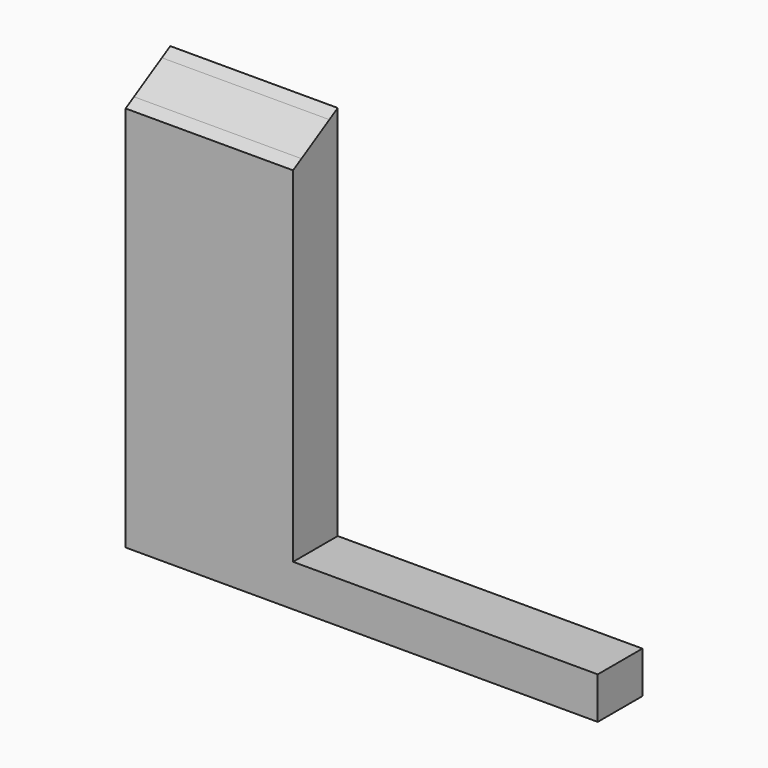
from build123d import *

# Parameters (mm, degrees)
F0_W     = 20
F0_H     = 50
F0_H_2   = 2
F1_DEPTH = 8
F3_DEPTH = 50
F4_DEPTH = 25.4
F5_T     = -2
F6_W     = 2
F6_H     = 4
F6_H_2   = 2
F6_W_2   = 20
F6_W_3   = 43.6544959545
F7_DEPTH = 8


with BuildPart() as f1:
    # F0 (on Front) → F1 (new body)
    with BuildSketch(Plane.XZ):
        Polygon((12, 27), (-12, 27), (-12, -27), (-10, -27), (-10, -25), (-10, 25), (10, 25), (10, -25), (10, -27), (12, -27), align=None)
        Rectangle(F0_W, F0_H)
        with Locations((0, -26)):
            Rectangle(F0_W, F0_H_2)
    extrude(amount=F1_DEPTH)

    # F2 (on Right) → F3 (cut)
    with BuildSketch(Plane.YZ):
        Polygon((-6.5, 23.2472232503), (-1.5, 26.1339745962), (0, 27), (-8, 27), (-8, 22.3811978465), align=None)
    extrude(amount=-F3_DEPTH, mode=Mode.SUBTRACT)

    # F2 (on Right) → F4 (cut)
    with BuildSketch(Plane.YZ):
        Polygon((-6.5, 23.2472232503), (-1.5, 26.1339745962), (0, 27), (-8, 27), (-8, 22.3811978465), align=None)
    extrude(amount=F4_DEPTH, mode=Mode.SUBTRACT)

    # F5
    f5_openings = [f1.faces().sort_by_distance(p)[0] for p in [
        (0, 0, 0),
        (0, -4, -27),
    ]]
    offset(amount=F5_T, openings=f5_openings)

    # F6 (on face) → F7 (join)
    with BuildSketch(Plane(origin=(0, 0, 0), x_dir=(-1, 0, 0), z_dir=(0, 1, 0))):
        with Locations((11, -29)):
            Rectangle(F6_W, F6_H)
        with Locations((11, -32)):
            Rectangle(F6_W, F6_H_2)
        Polygon((10, -31), (10, -27), (-10, -27), (-10, -29), (-53.6544959545, -29), (-53.6544959545, -31), (-10, -31), align=None)
        with Locations((0, -32)):
            Rectangle(F6_W_2, F6_H_2)
        Polygon((-10, -29), (-10, -27), (-12, -27), (-53.6544959545, -27), (-53.6544959545, -29), align=None)
        with Locations((-31.8272479773, -32)):
            Rectangle(F6_W_3, F6_H_2)
        with Locations((-54.6544959545, -32)):
            Rectangle(F6_W, F6_H_2)
        with Locations((-54.6544959545, -30)):
            Rectangle(F6_W, F6_H_2)
        with Locations((-54.6544959545, -28)):
            Rectangle(F6_W, F6_H_2)
    extrude(amount=-F7_DEPTH)


solid = f1.part
